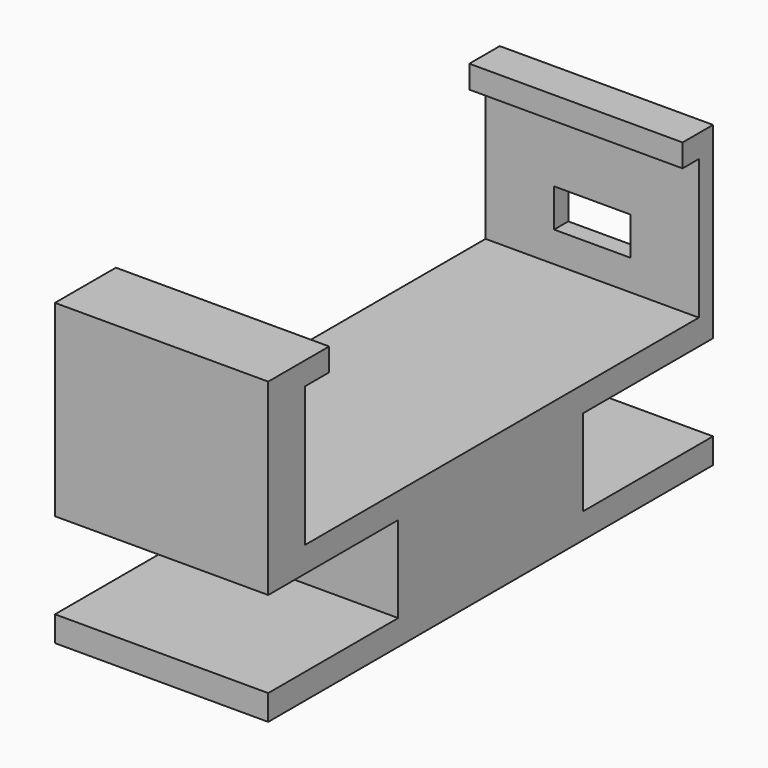
from build123d import *

# Parameters (mm, degrees)
F0_W      = 42
F0_H      = 109.5
F1_DEPTH  = 5
F2_W      = 42
F2_H      = 7.5
F2_H_2    = 15
F3_DEPTH  = 32
F4_W      = 42
F4_H      = 27.5
F5_DEPTH  = 4
F6_W      = 42
F6_H      = 27.5
F7_DEPTH  = 6
F8_W      = 15
F8_H      = 7.5
F9_DEPTH  = 3.501
F10_W     = 42
F10_H     = 54.75
F11_DEPTH = 22
F12_W     = 42
F12_H     = 17
F13_DEPTH = 32
F14_W     = 42
F14_H     = 17
F15_DEPTH = 32
F17_DEPTH = 1


# Not quite as in the source:
# - a feature names something its author has since deleted; it is built from what else it names


with BuildPart() as f1:
    # F0 (on Top) → F1 (new body)
    with BuildSketch(Plane.XY):
        Rectangle(F0_W, F0_H)
    extrude(amount=F1_DEPTH)

    # F2 (on face) → F3 (join)
    with BuildSketch(Plane.XY.offset(5)):
        with Locations((0, 51)):
            Rectangle(F2_W, F2_H)
        with Locations((0, -47.25)):
            Rectangle(F2_W, F2_H_2)
    extrude(amount=F3_DEPTH)

    # F4 (on face) → F5 (cut)
    with BuildSketch(Plane.XZ.offset(-47.25)):
        with Locations((0, 18.75)):
            Rectangle(F4_W, F4_H)
    extrude(amount=-F5_DEPTH, mode=Mode.SUBTRACT)

    # F6 (on face) → F7 (cut)
    with BuildSketch(Plane(origin=(0, -39.75, 0), x_dir=(-1, 0, 0), z_dir=(0, 1, 0))):
        with Locations((0, 18.75)):
            Rectangle(F6_W, F6_H)
    extrude(amount=-F7_DEPTH, mode=Mode.SUBTRACT)

    # F8 (on face) → F9 (cut, through all)
    with BuildSketch(Plane.XZ.offset(-51.25)):
        with Locations((0, 14.75)):
            Rectangle(F8_W, F8_H)
    extrude(amount=-F9_DEPTH, mode=Mode.SUBTRACT)

    # F10 (on face) → F11 (join)
    with BuildSketch(Plane(origin=(0, 0, 0), x_dir=(1, 0, 0), z_dir=(0, 0, -1))):
        with Locations((0, -27.375)):
            Rectangle(F10_W, F10_H)
        with Locations((0, 27.375)):
            Rectangle(F10_W, F10_H)
    extrude(amount=F11_DEPTH)

    # F12 (on face) → F13 (cut)
    with BuildSketch(Plane(origin=(0, 54.75, 0), x_dir=(-1, 0, 0), z_dir=(0, 1, 0))):
        with Locations((0, -8.5)):
            Rectangle(F12_W, F12_H)
    extrude(amount=-F13_DEPTH, mode=Mode.SUBTRACT)

    # F14 (on face) → F15 (cut)
    with BuildSketch(Plane.XZ.offset(54.75)):
        with Locations((0, -8.5)):
            Rectangle(F14_W, F14_H)
    extrude(amount=-F15_DEPTH, mode=Mode.SUBTRACT)

    # F16 (on face) → F17 (join)
    with BuildSketch(Plane(origin=(0, 54.75, 0), x_dir=(-1, 0, 0), z_dir=(0, 1, 0))):
        with BuildLine():
            ThreePointArc((9.9006995692, 9.0004714316), (13.1670561221, 1.352687349), (19.7461517383, 6.4392566621))
            ThreePointArc((19.7461517383, 6.4392566621), (19.5019885984, 8.0225954525), (18.7921845523, 9.458825093))
            ThreePointArc((18.7921845523, 9.458825093), (14.575302704, 11.6944347601), (10.2883124178, 9.5963982037))
            add(Edge.make_bspline(
                [(9.9006995692, 9.0004714316), (10.0318943543, 9.2081460376), (10.1611439812, 9.4065291941), (10.2883124178, 9.5963982037)],
                knots=[0, 0, 0, 0, 0.0231761706, 0.0231761706, 0.0231761706, 0.0231761706], degree=3))
        make_face()
        with BuildLine():
            add(Edge.make_bspline(
                [(12.5148005536, 5.2476986911), (11.5117744305, 4.2282460665), (10.7037792288, 2.9078259209), (13.5031697151, 2.0462179781), (14.5618504929, 1.8354499162)],
                knots=[0, 0, 0, 0, 0.4579310006, 1, 1, 1, 1], degree=3))
            add(Edge.make_bspline(
                [(13.5659415486, 4.241716412), (12.8136013619, 4.2865276682), (12.6872834074, 4.7459304754), (12.5148005536, 5.2476986911)],
                knots=[0, 0, 0, 0, 1.4549562665, 1.4549562665, 1.4549562665, 1.4549562665], degree=3))
            add(Edge.make_bspline(
                [(14.5618504929, 1.8354499162), (14.5289066888, 1.9808173354), (13.3458541311, 2.6761364671), (13.5659415486, 4.241716412)],
                knots=[0, 0, 0, 0, 2.604218323, 2.604218323, 2.604218323, 2.604218323], degree=3))
        make_face(mode=Mode.SUBTRACT)
        Polygon((13.47238521, 7.6377728132), (14.4902859979, 7.2816363839), (14.4902859979, 9.0213598503), (15.3866174204, 5.9906424503), (14.4902859979, 6.4392566621), (14.4902859979, 4.5215808953), align=None, mode=Mode.SUBTRACT)
        with BuildLine():
            add(Edge.make_bspline(
                [(15.4229601255, 4.1801771125), (16.5064311467, 3.1538456327), (16.8590547707, 1.9119603138), (18.5636819849, 4.2745726241), (19.0433704887, 5.2473602224)],
                knots=[0, 0, 0, 0, 0.4553347248, 1, 1, 1, 1], degree=3))
            add(Edge.make_bspline(
                [(16.4662250147, 5.1379367456), (16.2283618655, 4.4227829667), (15.8584250881, 4.3158873473), (15.4229601255, 4.1801771125)],
                knots=[0, 0, 0, 0, 1.4162291989, 1.4162291989, 1.4162291989, 1.4162291989], degree=3))
            add(Edge.make_bspline(
                [(19.0433704887, 5.2473602224), (18.3244173567, 4.9723164216), (17.3367887913, 4.1913386793), (16.4662250147, 5.1379367456)],
                knots=[0, 0, 0, 0, 2.5794674433, 2.5794674433, 2.5794674433, 2.5794674433], degree=3))
        make_face(mode=Mode.SUBTRACT)
        with BuildLine():
            add(Edge.make_bspline(
                [(13.5878011524, 9.0213598503), (13.0643112241, 9.5784787958), (11.4580836083, 10.9555165738), (10.5407517819, 8.58324464), (10.0999996066, 7.6000010595)],
                knots=[0, 0, 0, 0, 0.4589082861, 1, 1, 1, 1], degree=3))
            add(Edge.make_bspline(
                [(12.7311412425, 7.7330306741), (12.9425972845, 8.4564324625), (13.1576102672, 8.8697590463), (13.5878011524, 9.0213598503)],
                knots=[0, 0, 0, 0, 1.5471451992, 1.5471451992, 1.5471451992, 1.5471451992], degree=3))
            add(Edge.make_bspline(
                [(10.0999996066, 7.6000010595), (10.8170407506, 7.9740767086), (12.6145526151, 8.968960396), (12.7311412425, 7.7330306741)],
                knots=[0, 0, 0, 0, 2.5509056967, 2.5509056967, 2.5509056967, 2.5509056967], degree=3))
        make_face(mode=Mode.SUBTRACT)
        with BuildLine():
            add(Edge.make_bspline(
                [(16.3422210337, 7.7180123234), (17.2475090665, 8.9627835512), (18.0662711639, 9.9191930916), (15.3852159818, 10.9699756355), (14.4902859979, 10.9392784796)],
                knots=[0, 0, 0, 0, 0.4716209514, 1, 1, 1, 1], degree=3))
            add(Edge.make_bspline(
                [(15.403256887, 9.0213598503), (15.9476549795, 8.7934285242), (16.1248632097, 8.3395995036), (16.3422210337, 7.7180123234)],
                knots=[0, 0, 0, 0, 1.6063525282, 1.6063525282, 1.6063525282, 1.6063525282], degree=3))
            add(Edge.make_bspline(
                [(14.4902859979, 10.9392784796), (15.2978175145, 10.325451744), (15.8282139034, 9.1764941327), (15.403256887, 9.0213598503)],
                knots=[0, 0, 0, 0, 2.1241298719, 2.1241298719, 2.1241298719, 2.1241298719], degree=3))
        make_face(mode=Mode.SUBTRACT)
        with BuildLine():
            ThreePointArc((10.2883124178, 9.5963982037), (14.575302704, 11.6944347601), (18.7921845523, 9.458825093))
            add(Edge.make_bspline(
                [(10.2883124178, 9.5963982037), (12.0270262465, 12.1923872829), (14.0912584145, 13.7285191545), (14.5502114191, 17.0414015202), (15.1068634627, 13.6426153488), (16.9710466455, 12.3841964531), (18.7921845523, 9.458825093)],
                knots=[0.0231761706, 0.0231761706, 0.0231761706, 0.0231761706, 0.3400529794, 0.5078220439, 0.6757544935, 1, 1, 1, 1], degree=3))
        make_face()
        with BuildLine():
            ThreePointArc((10.2883124178, 9.5963982037), (10.0844189973, 9.3049957736), (9.9006995692, 9.0004714316))
            add(Edge.make_bspline(
                [(9.9006995692, 9.0004714316), (10.0318943543, 9.2081460376), (10.1611439812, 9.4065291941), (10.2883124178, 9.5963982037)],
                knots=[0, 0, 0, 0, 0.0231761706, 0.0231761706, 0.0231761706, 0.0231761706], degree=3))
        make_face()
    extrude(amount=F17_DEPTH)


solid = f1.part
